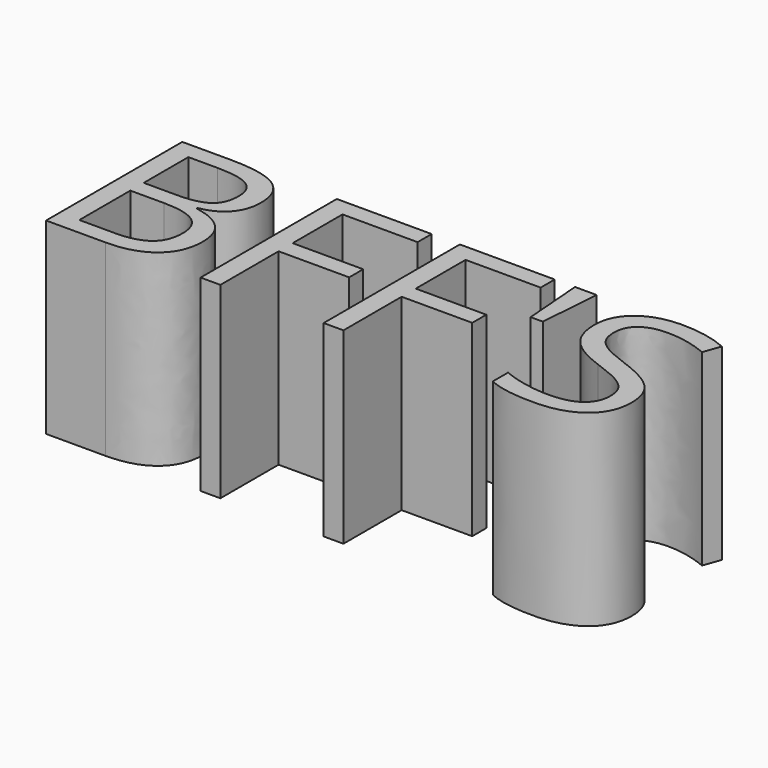
from build123d import *

# Parameters (mm, degrees)
F0_TEXT_SIZE = 32.234729992
F1_DEPTH     = 25.4


# Not quite as in the source:
# - Text() gives the source's letters only with a copy of the font that has no kerning and outlines rounded to 1/6400 em; it was checked with that copy


with BuildPart() as f1:
    # F0 (on Top) → F1 (new body)
    with BuildSketch(Plane.XY):
        with Locations((-42.6007444039, -9.924900718)):
            Text("BFF'S", F0_TEXT_SIZE, font='Open Sans', text_align=(TextAlign.LEFT, TextAlign.BOTTOM))
    extrude(amount=F1_DEPTH)


solid = f1.part
